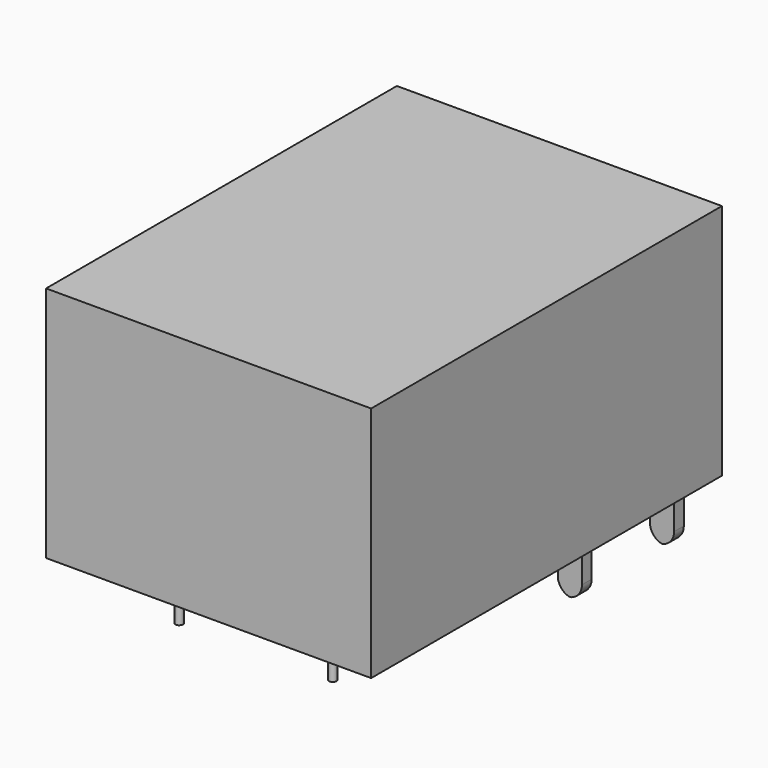
from build123d import *

# Parameters (mm, degrees)
F0_W        = 21.5
F0_H        = 29
F1_DEPTH    = 15.7
F2_W        = 1.6
F2_H        = 0.8
F2_R        = 0.25
F2_W_2      = 0.8
F2_H_2      = 1.6
F3_DEPTH    = 3.75
F4_T1_DEPTH = 5.8
F4_T3_DEPTH = 5.8
F4_T5_DEPTH = 5.8


# Not quite as in the source:
# - a fillet or chamfer that OpenCascade refuses, or shapes differently, is made with other operations: its cross-section is extruded or revolved along the edge and cut away or added


with BuildPart() as f1:
    # F0 (on Top) → F1 (new body)
    with BuildSketch(Plane.XY):
        Rectangle(F0_W, F0_H)
    extrude(amount=F1_DEPTH)

    # F2 (on face) → F3 (join)
    with BuildSketch(Plane.XY):
        with Locations((8.63, 12.6)):
            Rectangle(F2_W, F2_H)
        with Locations((8.63, 4.98)):
            Rectangle(F2_W, F2_H)
        with Locations((-5.34, -10.26)):
            Circle(F2_R)
        with Locations((4.82, -10.26)):
            Circle(F2_R)
        with Locations((-9.15, 2.44)):
            Rectangle(F2_W_2, F2_H_2)
    extrude(amount=-F3_DEPTH)

    # F4: fillet of radius 1 on 6 edges, made by hand

    # F4_s2 → F4_t1 (cut)
    with BuildSketch(Plane.XZ.offset(-15.5)):
        with BuildLine():
            ThreePointArc((7.83, -2.75), (8.1228932188, -3.4571067812), (8.83, -3.75))
            Line((8.83, -3.75), (7.83, -3.75))
            Line((7.83, -3.75), (7.83, -2.75))
        make_face()
        with BuildLine():
            ThreePointArc((9.43, -2.75), (9.1371067812, -3.4571067812), (8.43, -3.75))
            Line((8.43, -3.75), (9.43, -3.75))
            Line((9.43, -3.75), (9.43, -2.75))
        make_face()
    extrude(amount=F4_T1_DEPTH, mode=Mode.SUBTRACT)

    # F4_s4 → F4_t3 (cut)
    with BuildSketch(Plane.XZ.offset(-7.88)):
        with BuildLine():
            ThreePointArc((7.83, -2.75), (8.1228932188, -3.4571067812), (8.83, -3.75))
            Line((8.83, -3.75), (7.83, -3.75))
            Line((7.83, -3.75), (7.83, -2.75))
        make_face()
        with BuildLine():
            ThreePointArc((9.43, -2.75), (9.1371067812, -3.4571067812), (8.43, -3.75))
            Line((8.43, -3.75), (9.43, -3.75))
            Line((9.43, -3.75), (9.43, -2.75))
        make_face()
    extrude(amount=F4_T3_DEPTH, mode=Mode.SUBTRACT)

    # F4_s6 → F4_t5 (cut)
    with BuildSketch(Plane.YZ.offset(-12.05)):
        with BuildLine():
            ThreePointArc((1.64, -2.75), (1.9328932188, -3.4571067812), (2.64, -3.75))
            Line((2.64, -3.75), (1.64, -3.75))
            Line((1.64, -3.75), (1.64, -2.75))
        make_face()
        with BuildLine():
            ThreePointArc((3.24, -2.75), (2.9471067812, -3.4571067812), (2.24, -3.75))
            Line((2.24, -3.75), (3.24, -3.75))
            Line((3.24, -3.75), (3.24, -2.75))
        make_face()
    extrude(amount=F4_T5_DEPTH, mode=Mode.SUBTRACT)


solid = f1.part
